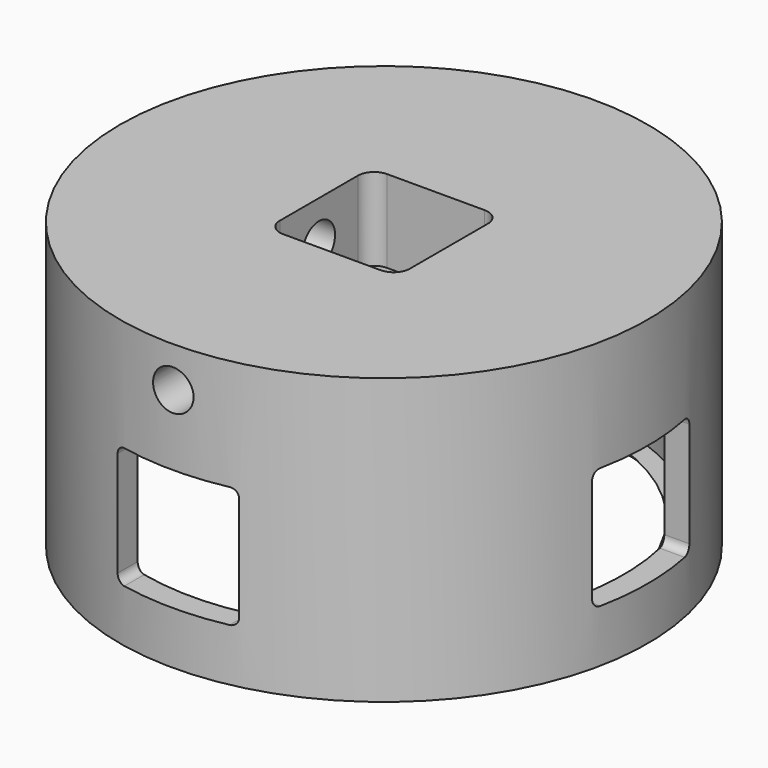
from build123d import *

# Parameters (mm, degrees)
F3_DEPTH        = 25
F4_R            = 2.5
F5_DEPTH        = 24.571
F5_COPIES_COUNT = 2
F5_COPIES_ANGLE = 90
F7_DEPTH        = 32.6010001
F7_COPIES_COUNT = 4


# Not quite as in the source:
# - a pattern or mirror of a feature is missing from the dataset's text; its kind, count and spacing are read off the source's solid


with BuildPart() as f1:
    # F0 (on Front) → F1 (revolve)
    with BuildSketch(Plane.XZ):
        Polygon((0, -10.2), (0, 0), (-32.6, 0), (-32.6, -35.2), (-30.25, -35.2), (-27.25, -32.2), (-29.6, -32.2), (-29.6, -10.2), align=None)
    revolve(axis=Axis((0, 0, -5.1), (0, 0, 1)))

    # F2 (on face) → F3 (cut)
    with BuildSketch(Plane.XY):
        with BuildLine():
            ThreePointArc((8.03, 6.03), (7.4442135624, 7.4442135624), (6.03, 8.03))
            Line((6.03, 8.03), (-6.03, 8.03))
            ThreePointArc((-6.03, 8.03), (-7.4442135624, 7.4442135624), (-8.03, 6.03))
            Line((-8.03, 6.03), (-8.03, -6.03))
            ThreePointArc((-8.03, -6.03), (-7.4442135624, -7.4442135624), (-6.03, -8.03))
            Line((-6.03, -8.03), (6.03, -8.03))
            ThreePointArc((6.03, -8.03), (7.4442135624, -7.4442135624), (8.03, -6.03))
            Line((8.03, -6.03), (8.03, 6.03))
        make_face()
    extrude(amount=-F3_DEPTH, mode=Mode.SUBTRACT)

    # F4 (on face) → F5 (cut, through all)
    with BuildSketch(Plane.YZ.offset(-8.03)):
        with Locations((0, -5)):
            Circle(F4_R)
    f5 = extrude(amount=-F5_DEPTH, mode=Mode.SUBTRACT)

    # F5_copies: F5 ×2 about axis
    f5_copies_axis = Axis((0, 0, 0), (0, 0, 1))
    for i in range(1, F5_COPIES_COUNT):
        add(f5.rotate(f5_copies_axis, i * F5_COPIES_ANGLE / (F5_COPIES_COUNT - 1)), mode=Mode.SUBTRACT)

    # F6 (on Front) → F7 (cut, through all)
    with BuildSketch(Plane.XZ):
        with BuildLine():
            ThreePointArc((-7.5, -27.7), (-7.2071067812, -28.4071067812), (-6.5, -28.7))
            Line((-6.5, -28.7), (6.5, -28.7))
            ThreePointArc((6.5, -28.7), (7.2071067812, -28.4071067812), (7.5, -27.7))
            Line((7.5, -27.7), (7.5, -14.7))
            ThreePointArc((7.5, -14.7), (7.2071067812, -13.9928932188), (6.5, -13.7))
            Line((6.5, -13.7), (-6.5, -13.7))
            ThreePointArc((-6.5, -13.7), (-7.2071067812, -13.9928932188), (-7.5, -14.7))
            Line((-7.5, -14.7), (-7.5, -27.7))
        make_face()
    f7 = extrude(amount=-F7_DEPTH, mode=Mode.SUBTRACT)

    # F7_copies: F7 ×4 about axis
    f7_copies_axis = Axis((0, 0, 0), (0, 0, 1))
    for i in range(1, F7_COPIES_COUNT):
        add(f7.rotate(f7_copies_axis, i * 360 / F7_COPIES_COUNT), mode=Mode.SUBTRACT)


solid = f1.part
